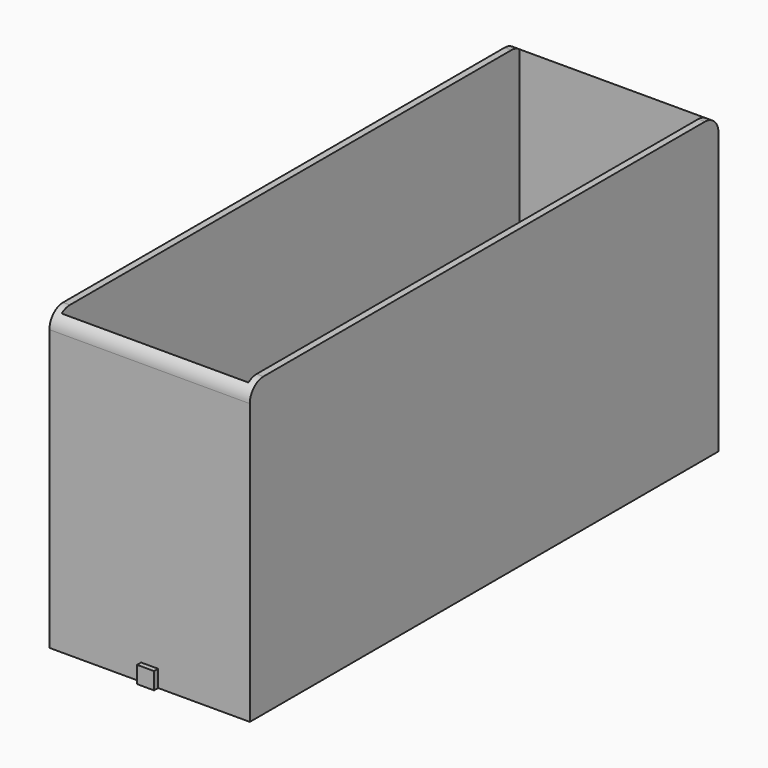
from build123d import *

# Parameters (mm, degrees)
F0_W        = 23.6
F0_H        = 69
F0_W_2      = 22
F0_H_2      = 67.4
F1_DEPTH    = 35
F2_T1_DEPTH = 33.6
F3_W        = 2
F3_H        = 0.6
F4_DEPTH    = 2


# Not quite as in the source:
# - a fillet or chamfer that OpenCascade refuses, or shapes differently, is made with other operations: its cross-section is extruded or revolved along the edge and cut away or added


with BuildPart() as f1:
    # F0 (on Top) → F1 (new body)
    with BuildSketch(Plane.XY):
        Rectangle(F0_W, F0_H)
        Rectangle(F0_W_2, F0_H_2, mode=Mode.SUBTRACT)
    extrude(amount=F1_DEPTH)

    # F2: fillet of radius 2 on 2 edges, made by hand

    # F2_s2 → F2_t1 (cut)
    with BuildSketch(Plane.YZ.offset(-16.8)):
        with BuildLine():
            ThreePointArc((-34.5, 33), (-33.9142135624, 34.4142135624), (-32.5, 35))
            Line((-32.5, 35), (-34.5, 35))
            Line((-34.5, 35), (-34.5, 33))
        make_face()
        with BuildLine():
            ThreePointArc((34.5, 33), (33.9142135624, 34.4142135624), (32.5, 35))
            Line((32.5, 35), (34.5, 35))
            Line((34.5, 35), (34.5, 33))
        make_face()
    extrude(amount=F2_T1_DEPTH, mode=Mode.SUBTRACT)

    # F3 (on face) → F4 (join)
    with BuildSketch(Plane(origin=(0, 0, 0), x_dir=(1, 0, 0), z_dir=(0, 0, -1))):
        with Locations((0, 34.8)):
            Rectangle(F3_W, F3_H)
        with Locations((0, -34.8)):
            Rectangle(F3_W, F3_H)
    extrude(amount=-F4_DEPTH)


solid = f1.part
